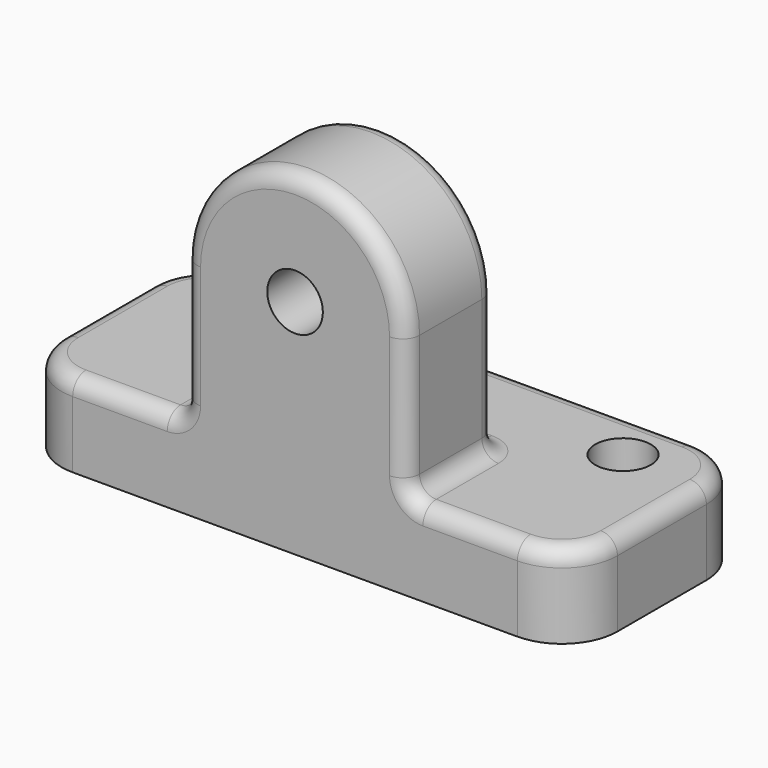
from build123d import *

# Parameters (mm, degrees)
F0_R     = 5
F0_W     = 40
F0_H     = 40
F1_DEPTH = 15
F2_R     = 5
F3_DEPTH = 20
F4_R     = 3


with BuildPart() as f1:
    # F0 (on Top) → F1 (new body)
    with BuildSketch(Plane.XY):
        with BuildLine():
            Line((-40, -20), (-20.3233100474, -20))
            Line((-20.3233100474, -20), (-20.3233100474, 20))
            Line((-20.3233100474, 20), (-40, 20))
            ThreePointArc((-40, 20), (-47.0710678119, 17.0710678119), (-50, 10))
            Line((-50, 10), (-50, -10))
            ThreePointArc((-50, -10), (-47.0710678119, -17.0710678119), (-40, -20))
        make_face()
        with Locations((-35, 10)):
            Circle(F0_R, mode=Mode.SUBTRACT)
        with Locations((-0.3233100474, 0)):
            Rectangle(F0_W, F0_H)
        with BuildLine():
            Line((19.6766899526, -20), (40, -20))
            ThreePointArc((40, -20), (47.0710678119, -17.0710678119), (50, -10))
            Line((50, -10), (50, 10))
            ThreePointArc((50, 10), (47.0710678119, 17.0710678119), (40, 20))
            Line((40, 20), (19.6766899526, 20))
            Line((19.6766899526, 20), (19.6766899526, -20))
        make_face()
        with Locations((35, 10)):
            Circle(F0_R, mode=Mode.SUBTRACT)
    extrude(amount=F1_DEPTH)

    # F2 (on face) → F3 (join)
    with BuildSketch(Plane.XZ.offset(20)):
        with BuildLine():
            ThreePointArc((20, 40), (0, 60), (-20, 40))
            Line((-20, 40), (-20, 15))
            Line((-20, 15), (20, 15))
            Line((20, 15), (20, 40))
        make_face()
        with Locations((0, 40)):
            Circle(F2_R, mode=Mode.SUBTRACT)
    extrude(amount=-F3_DEPTH)

    # F4
    f4_edges = [f1.edges().sort_by_distance(p)[0] for p in [
        (0, 0, 60),
        (0, 0, 15),
        (0, -20, 60),
        (-30, -20, 15),
        (-20, -20, 27.5),
        (20, -20, 27.5),
        (30, -20, 15),
        (-47.071068, -17.071068, 15),
        (47.071068, -17.071068, 15),
        (-50, 0, 15),
        (-47.071068, 17.071068, 15),
        (0, 20, 15),
        (47.071068, 17.071068, 15),
        (50, 0, 15),
        (20, -10, 15),
        (-20, -10, 15),
        (20, 0, 27.5),
        (-20, 0, 27.5),
    ]]
    fillet(f4_edges, radius=F4_R)


solid = f1.part
